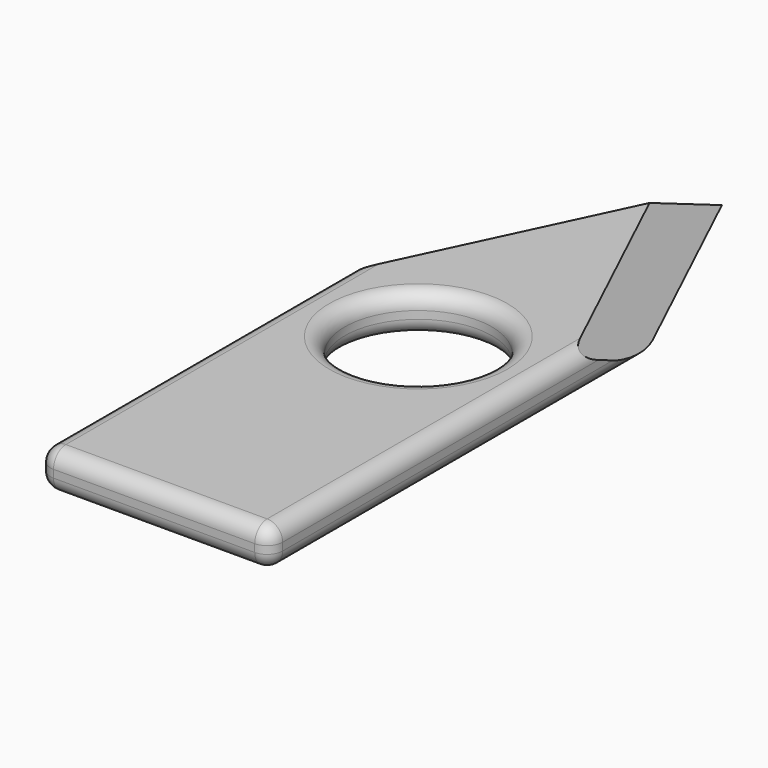
from build123d import *

# Parameters (mm, degrees)
F0_W     = 30
F0_H     = 60
F0_R     = 9.5
F1_DEPTH = 5
F2_SIZE  = 4.99999
F3_R     = 2
F4_R     = 2


# Not quite as in the source:
# - a fillet or chamfer is up to 0.001 mm smaller than in the source, because OpenCascade refuses the exact size


with BuildPart() as f1:
    # F0 (on Top) → F1 (new body)
    with BuildSketch(Plane.XY):
        with Locations((0, -12.6652074978)):
            Rectangle(F0_W, F0_H)
        Circle(F0_R, mode=Mode.SUBTRACT)
        Polygon((-15, 17.3347925022), (15, 17.3347925022), (0, 49.0306541324), align=None)
    extrude(amount=F1_DEPTH)

    # F2 (size 5 in the source; OpenCascade refuses exactly that, so slightly less here)
    f2_edges = [f1.edges().sort_by_distance(p)[0] for p in [
        (-7.5, 33.182723, 5),
        (7.5, 33.182723, 5),
    ]]
    chamfer(f2_edges, length=F2_SIZE)

    # F3
    f3_edges = [f1.edges().sort_by_distance(p)[0] for p in [
        (-15, -18.509537, 5),
        (15, -18.509537, 5),
        (15, -12.665207, 0),
        (-15, -12.665207, 0),
        (-9.5, 0, 5),
        (-9.5, 0, 0),
    ]]
    fillet(f3_edges, radius=F3_R)

    # F4
    f4_edges = [f1.edges().sort_by_distance(p)[0] for p in [
        (0, -42.665207, 5),
    ]]
    fillet(f4_edges, radius=F4_R)


solid = f1.part
